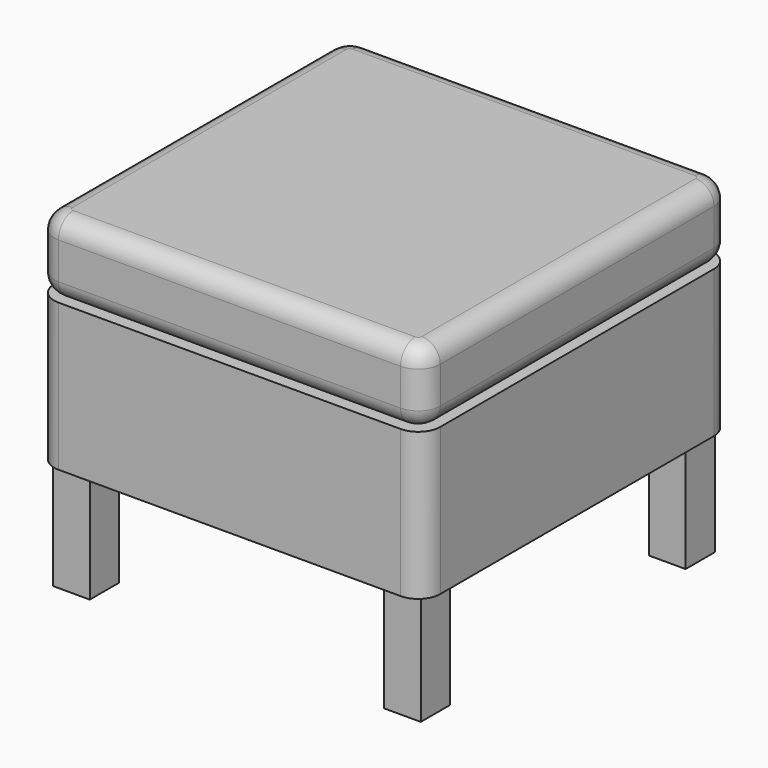
from build123d import *

# Parameters (mm, degrees)
F0_W          = 500
F0_H          = 500
F1_DEPTH      = 150
F2_W          = 400
F2_H          = 150
F3_DEPTH      = 500.001
F4_W          = 400
F4_H          = 150
F5_DEPTH      = 500.001
F6_W          = 400
F6_H          = 150
F7_DEPTH      = 500.001
F8_W          = 525
F8_H          = 525
F9_DEPTH      = 200
F11_W         = 525
F11_H         = 525
F12_DEPTH     = 100
F13_R         = 25
F14_R         = 25
F15_T1_DEPTH  = 100
F15_T4_ANGLE  = 90
F15_T6_ANGLE  = 90
F15_T8_ANGLE  = 90
F15_T10_ANGLE = 90
F15_T12_ANGLE = 90
F15_T14_ANGLE = 90
F15_T16_ANGLE = 90
F15_T18_ANGLE = 90
F15_2_F1_R    = 30
F15_2_F2_R    = 30
F15_2_F3_R    = 30
F15_2_F4_R    = 30


# Not quite as in the source:
# - a fillet or chamfer that OpenCascade refuses, or shapes differently, is made with other operations: its cross-section is extruded or revolved along the edge and cut away or added


with BuildPart() as f1:
    # F0 (on Top) → F1 (new body)
    with BuildSketch(Plane.XY):
        Rectangle(F0_W, F0_H)
    extrude(amount=-F1_DEPTH)

    # F2 (on face) → F3 (cut, through all)
    with BuildSketch(Plane.XZ.offset(250)):
        with Locations((0, -75)):
            Rectangle(F2_W, F2_H)
    extrude(amount=-F3_DEPTH, mode=Mode.SUBTRACT)

    # F4 (on face) → F5 (cut, through all)
    with BuildSketch(Plane(origin=(-250, 0, 0), x_dir=(0, -1, 0), z_dir=(-1, 0, 0))):
        with Locations((0, -75)):
            Rectangle(F4_W, F4_H)
    extrude(amount=-F5_DEPTH, mode=Mode.SUBTRACT)

    # F6 (on face) → F7 (cut, through all)
    with BuildSketch(Plane.YZ.offset(250)):
        with Locations((0, -75)):
            Rectangle(F6_W, F6_H)
    extrude(amount=-F7_DEPTH, mode=Mode.SUBTRACT)


with BuildPart() as f9:
    # F8 (on Top) → F9 (new body)
    with BuildSketch(Plane.XY):
        Rectangle(F8_W, F8_H)
    extrude(amount=F9_DEPTH)

    # F15#2: fillet of radius 30 on 4 edges, made by hand

    # F15_2_f1
    f15_2_f1_edges = [f9.edges().sort_by_distance(p)[0] for p in [
        (-262.5, 262.5, 100),
    ]]
    fillet(f15_2_f1_edges, radius=F15_2_F1_R)

    # F15_2_f2
    f15_2_f2_edges = [f9.edges().sort_by_distance(p)[0] for p in [
        (-262.5, -262.5, 100),
    ]]
    fillet(f15_2_f2_edges, radius=F15_2_F2_R)

    # F15_2_f3
    f15_2_f3_edges = [f9.edges().sort_by_distance(p)[0] for p in [
        (262.5, -262.5, 100),
    ]]
    fillet(f15_2_f3_edges, radius=F15_2_F3_R)

    # F15_2_f4
    f15_2_f4_edges = [f9.edges().sort_by_distance(p)[0] for p in [
        (262.5, 262.5, 100),
    ]]
    fillet(f15_2_f4_edges, radius=F15_2_F4_R)


with BuildPart() as f12:
    # F11 (on face) → F12 (new body)
    with BuildSketch(Plane.XY.offset(200)):
        Rectangle(F11_W, F11_H)
    extrude(amount=F12_DEPTH)

    # F13
    f13_edges = [f12.edges().sort_by_distance(p)[0] for p in [
        (0, 262.5, 200),
        (262.5, 0, 200),
        (-262.5, 0, 200),
        (0, -262.5, 200),
    ]]
    fillet(f13_edges, radius=F13_R)

    # F14
    f14_edges = [f12.edges().sort_by_distance(p)[0] for p in [
        (0, 262.5, 300),
        (262.5, 0, 300),
        (-262.5, 0, 300),
        (0, -262.5, 300),
    ]]
    fillet(f14_edges, radius=F14_R)

    # F15: fillet of radius 30 on 4 edges, made by hand

    # F15_s2 → F15_t1 (cut)
    with BuildSketch(Plane.XY.offset(200)):
        with BuildLine():
            ThreePointArc((-232.5, 262.5), (-253.7132034356, 253.7132034356), (-262.5, 232.5))
            Line((-262.5, 232.5), (-262.5, 262.5))
            Line((-262.5, 262.5), (-232.5, 262.5))
        make_face()
        with BuildLine():
            ThreePointArc((232.5, 262.5), (253.7132034356, 253.7132034356), (262.5, 232.5))
            Line((262.5, 232.5), (262.5, 262.5))
            Line((262.5, 262.5), (232.5, 262.5))
        make_face()
        with BuildLine():
            ThreePointArc((262.5, -232.5), (253.7132034356, -253.7132034356), (232.5, -262.5))
            Line((232.5, -262.5), (262.5, -262.5))
            Line((262.5, -262.5), (262.5, -232.5))
        make_face()
        with BuildLine():
            ThreePointArc((-262.5, -232.5), (-253.7132034356, -253.7132034356), (-232.5, -262.5))
            Line((-232.5, -262.5), (-262.5, -262.5))
            Line((-262.5, -262.5), (-262.5, -232.5))
        make_face()
    extrude(amount=F15_T1_DEPTH, mode=Mode.SUBTRACT)

    # F15_s3 → F15_t4 (revolve, cut)
    with BuildSketch(Plane.YZ.offset(-232.5)):
        with BuildLine():
            ThreePointArc((-237.5, 200), (-255.1776695297, 207.3223304703), (-262.5, 225))
            Line((-262.5, 225), (-262.5, 200))
            Line((-262.5, 200), (-237.5, 200))
        make_face()
    revolve(axis=Axis((-232.5, -232.5, 200), (0, 0, -1)), revolution_arc=F15_T4_ANGLE, mode=Mode.SUBTRACT)

    # F15_s5 → F15_t6 (revolve, cut)
    with BuildSketch(Plane.XZ.offset(232.5)):
        with BuildLine():
            ThreePointArc((-237.5, 300), (-255.1776695297, 292.6776695297), (-262.5, 275))
            Line((-262.5, 275), (-262.5, 300))
            Line((-262.5, 300), (-237.5, 300))
        make_face()
    revolve(axis=Axis((-232.5, -232.5, 300), (0, 0, 1)), revolution_arc=F15_T6_ANGLE, mode=Mode.SUBTRACT)

    # F15_s7 → F15_t8 (revolve, cut)
    with BuildSketch(Plane.XZ.offset(232.5)):
        with BuildLine():
            ThreePointArc((237.5, 200), (255.1776695297, 207.3223304703), (262.5, 225))
            Line((262.5, 225), (262.5, 200))
            Line((262.5, 200), (237.5, 200))
        make_face()
    revolve(axis=Axis((232.5, -232.5, 200), (0, 0, -1)), revolution_arc=F15_T8_ANGLE, mode=Mode.SUBTRACT)

    # F15_s9 → F15_t10 (revolve, cut)
    with BuildSketch(Plane.YZ.offset(232.5)):
        with BuildLine():
            ThreePointArc((-237.5, 300), (-255.1776695297, 292.6776695297), (-262.5, 275))
            Line((-262.5, 275), (-262.5, 300))
            Line((-262.5, 300), (-237.5, 300))
        make_face()
    revolve(axis=Axis((232.5, -232.5, 300), (0, 0, 1)), revolution_arc=F15_T10_ANGLE, mode=Mode.SUBTRACT)

    # F15_s11 → F15_t12 (revolve, cut)
    with BuildSketch(Plane.YZ.offset(232.5)):
        with BuildLine():
            ThreePointArc((237.5, 200), (255.1776695297, 207.3223304703), (262.5, 225))
            Line((262.5, 225), (262.5, 200))
            Line((262.5, 200), (237.5, 200))
        make_face()
    revolve(axis=Axis((232.5, 232.5, 200), (0, 0, -1)), revolution_arc=F15_T12_ANGLE, mode=Mode.SUBTRACT)

    # F15_s13 → F15_t14 (revolve, cut)
    with BuildSketch(Plane.XZ.offset(-232.5)):
        with BuildLine():
            ThreePointArc((237.5, 300), (255.1776695297, 292.6776695297), (262.5, 275))
            Line((262.5, 275), (262.5, 300))
            Line((262.5, 300), (237.5, 300))
        make_face()
    revolve(axis=Axis((232.5, 232.5, 300), (0, 0, 1)), revolution_arc=F15_T14_ANGLE, mode=Mode.SUBTRACT)

    # F15_s15 → F15_t16 (revolve, cut)
    with BuildSketch(Plane.XZ.offset(-232.5)):
        with BuildLine():
            ThreePointArc((-237.5, 200), (-255.1776695297, 207.3223304703), (-262.5, 225))
            Line((-262.5, 225), (-262.5, 200))
            Line((-262.5, 200), (-237.5, 200))
        make_face()
    revolve(axis=Axis((-232.5, 232.5, 200), (0, 0, -1)), revolution_arc=F15_T16_ANGLE, mode=Mode.SUBTRACT)

    # F15_s17 → F15_t18 (revolve, cut)
    with BuildSketch(Plane.YZ.offset(-232.5)):
        with BuildLine():
            ThreePointArc((237.5, 300), (255.1776695297, 292.6776695297), (262.5, 275))
            Line((262.5, 275), (262.5, 300))
            Line((262.5, 300), (237.5, 300))
        make_face()
    revolve(axis=Axis((-232.5, 232.5, 300), (0, 0, 1)), revolution_arc=F15_T18_ANGLE, mode=Mode.SUBTRACT)


solid = Compound([f1.part, f9.part, f12.part])
